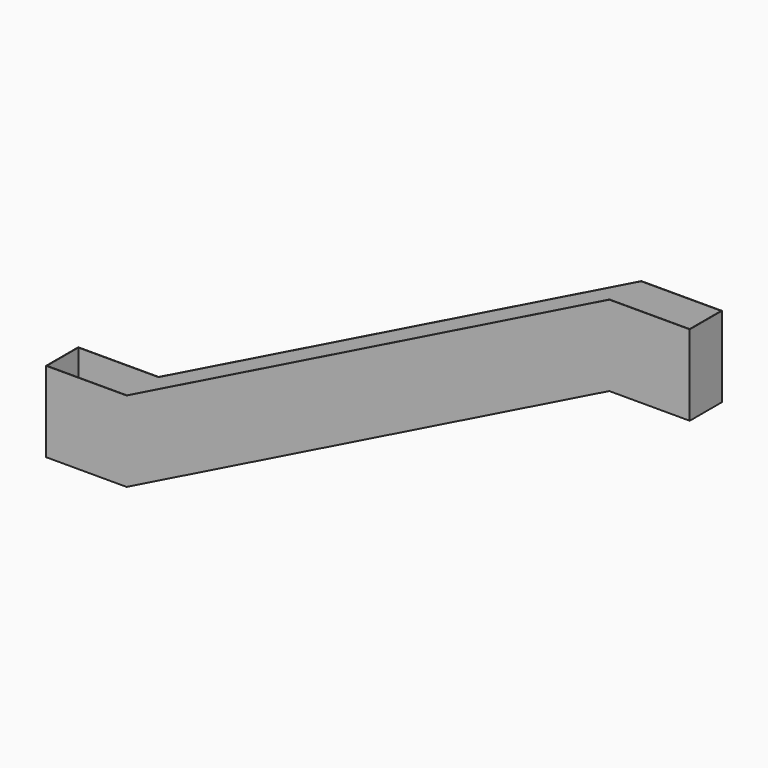
from build123d import *

# Parameters (mm, degrees)
F1_DEPTH = 100
F2_T     = -1
F5_D     = 20


# Not quite as in the source:
# - the program builds the solid bodies; features that only make, move or delete a surface that nothing else refers to are left out


with BuildPart() as f1:
    # F0 (on Front) → F1 (new body)
    with BuildSketch(Plane.XZ):
        Polygon((0, 200), (0, 0), (200, 0), (1400, 600), (1600, 600), (1600, 800), (1400, 800), (200, 200), align=None)
    extrude(amount=F1_DEPTH)

    # F2
    f2_openings = [f1.faces().sort_by_distance(p)[0] for p in [
        (100, -50, 200),
        (1500, -50, 800),
        (800, -50, 500),
    ]]
    offset(amount=F2_T, openings=f2_openings, kind=Kind.INTERSECTION)

    # F5 (through all)
    with Locations(Plane.XY.offset(601)):
        with Locations((1587, -13), (1587, -87)):
            Hole(F5_D / 2)


solid = f1.part
